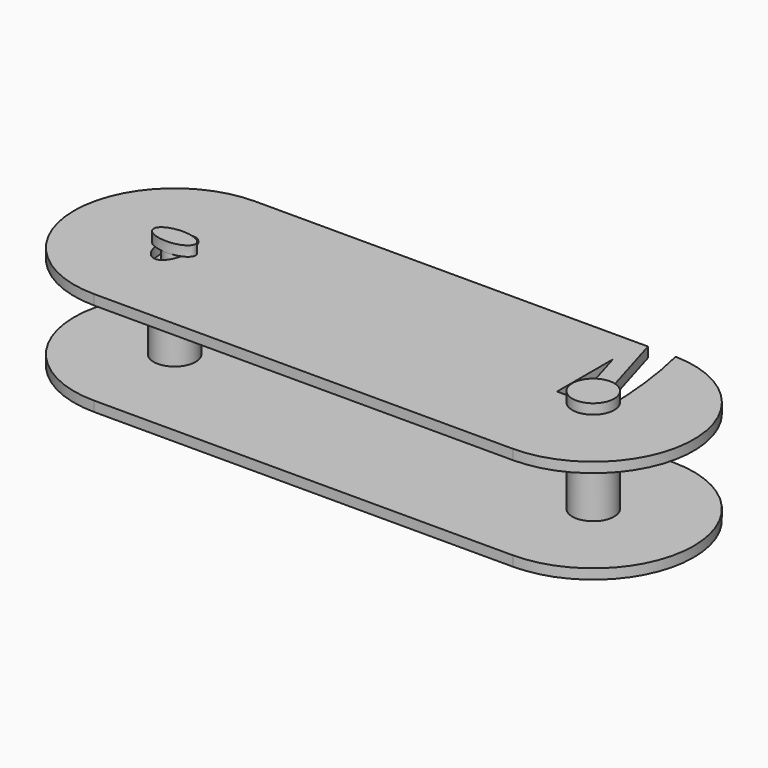
from build123d import *

# Parameters (mm, degrees)
F1_DEPTH  = 1.2
F2_R      = 2.5
F3_DEPTH  = 10
F4_R      = 1.25
F5_R      = 1.25
F6_DEPTH  = 1.2
F8_R      = 2.5
F8_R_2    = 1.25
F9_DEPTH  = 1.2
F11_DEPTH = 1.2


with BuildPart() as f1:
    # F0 (on Top) → F1 (new body)
    with BuildSketch(Plane.XY):
        with BuildLine():
            ThreePointArc((0, 12), (-12, 0), (0, -12))
            Line((0, -12), (50, -12))
            ThreePointArc((50, -12), (62, 0), (50, 12))
            Line((50, 12), (0, 12))
        make_face()
    extrude(amount=F1_DEPTH)

    # F2 (on face) → F3 (join)
    with BuildSketch(Plane.XY.offset(1.2)):
        Circle(F2_R)
        with Locations((50, 0)):
            Circle(F2_R)
    extrude(amount=F3_DEPTH)

    # F4 (on face) + F5 (on face) → F6 (join)
    with BuildSketch(Plane.XY.offset(11.2)):
        Circle(F4_R)
    with BuildSketch(Plane.XY.offset(11.2)):
        with Locations((50, 0)):
            Circle(F5_R)
    extrude(amount=F6_DEPTH)

    # F7 (on face) + F8 (on face) → F9 (join)
    with BuildSketch(Plane.XY.offset(12.4)):
        with BuildLine():
            add(Edge.make_bspline(
                [(4.2e-09, -1.25), (2.5000000021, -1.2499999979), (2.5, 1e-09), (2.4999999979, 1.25), (0, 1.25)],
                knots=[1.5707963285, 1.5707963285, 1.5707963285, 3.1415926544, 3.1415926544, 4.7123889804, 4.7123889804, 4.7123889804], degree=2, weights=[1, 0.7071067815, 1, 0.7071067815, 1]))
            ThreePointArc((0, 1.25), (0.8838834765, 0.8838834765), (1.25, 0))
            ThreePointArc((1.25, 0), (0.883883478, -0.883883475), (4.2e-09, -1.25))
        make_face()
        with BuildLine():
            ThreePointArc((1.25, 0), (0.8838834765, 0.8838834765), (0, 1.25))
            ThreePointArc((0, 1.25), (-1.25, -2.1e-09), (4.2e-09, -1.25))
            ThreePointArc((4.2e-09, -1.25), (0.883883478, -0.883883475), (1.25, 0))
        make_face()
        with BuildLine():
            ThreePointArc((4.2e-09, -1.25), (-1.25, -2.1e-09), (0, 1.25))
            add(Edge.make_bspline(
                [(0, 1.25), (-2.5000000021, 1.25), (-2.5, -1e-09), (-2.4999999979, -1.2500000021), (4.2e-09, -1.25)],
                knots=[4.7123889804, 4.7123889804, 4.7123889804, 6.283185308, 6.283185308, 7.8539816357, 7.8539816357, 7.8539816357], degree=2, weights=[1, 0.7071067809, 1, 0.7071067809, 1]))
        make_face()
    with BuildSketch(Plane.XY.offset(12.4)):
        with Locations((50, 0)):
            Circle(F8_R)
        with Locations((50, 0)):
            Circle(F8_R_2, mode=Mode.SUBTRACT)
        with Locations((50, 0)):
            Circle(F8_R_2)
    extrude(amount=F9_DEPTH)


with BuildPart() as f11:
    # F10 (on face) → F11 (new body)
    with BuildSketch(Plane.XY.offset(11.2)):
        with BuildLine():
            ThreePointArc((0, 12), (-12, 0), (0, -12))
            Line((0, -12), (50, -12))
            ThreePointArc((50, -12), (61.9994137232, -0.1186182953), (50.237225, 11.99765495))
            ThreePointArc((50.237225, 11.99765495), (51.2955903136, 6.0402743626), (51.65, 0))
            ThreePointArc((51.65, 0), (50.2015083771, -1.6376490387), (48.3992189406, -0.4))
            Line((48.3992189406, -0.4), (45.9992189406, -0.4))
            Line((45.9992189406, -0.4), (45.9992189406, 7.9439693035))
            Line((45.9992189406, 7.9439693035), (48.35, 0))
            ThreePointArc((48.35, 0), (48.833273811, 1.166726189), (50, 1.65))
            Line((50, 1.65), (46.9372258332, 12))
            Line((46.9372258332, 12), (0, 12))
        make_face()
        with BuildLine():
            add(Edge.make_bspline(
                [(1.0168341302, 2.2838669733), (0, 3.6823510732), (-1.0168341302, 2.2838669733)],
                knots=[5.6191964791, 5.6191964791, 5.6191964791, 6.9471741352, 6.9471741352, 6.9471741352], degree=2, weights=[1, 0.7875403356, 1]))
            ThreePointArc((1.0168341302, 2.2838669733), (2.0966741909, 1.3616010198), (2.5, 0))
            ThreePointArc((2.5, 0), (2.0966741909, -1.3616010198), (1.0168341302, -2.2838669733))
            add(Edge.make_bspline(
                [(-1.0168341302, -2.2838669733), (0, -3.6823510732), (1.0168341302, -2.2838669733)],
                knots=[2.4776038255, 2.4776038255, 2.4776038255, 3.8055814816, 3.8055814816, 3.8055814816], degree=2, weights=[1, 0.7875403356, 1]))
            ThreePointArc((-1.0168341302, -2.2838669733), (-2.5, 0), (-1.0168341302, 2.2838669733))
        make_face(mode=Mode.SUBTRACT)
        with BuildLine():
            add(Edge.make_bspline(
                [(1.65, 0), (1.65, 1.4130539516), (1.0168341302, 2.2838669733)],
                knots=[4.7123889804, 4.7123889804, 4.7123889804, 5.6191964791, 5.6191964791, 5.6191964791], degree=2, weights=[1, 0.8989613755, 1]))
            add(Edge.make_bspline(
                [(1.0168341302, -2.2838669733), (1.65, -1.4130539516), (1.65, 0)],
                knots=[3.8055814816, 3.8055814816, 3.8055814816, 4.7123889804, 4.7123889804, 4.7123889804], degree=2, weights=[1, 0.8989613755, 1]))
            ThreePointArc((1.0168341302, -2.2838669733), (2.0966741909, -1.3616010198), (2.5, 0))
            ThreePointArc((2.5, 0), (2.0966741909, 1.3616010198), (1.0168341302, 2.2838669733))
        make_face()
        with BuildLine():
            add(Edge.make_bspline(
                [(-1.0168341302, 2.2838669733), (-2.6774278313, 0), (-1.0168341302, -2.2838669733)],
                knots=[0.663988828, 0.663988828, 0.663988828, 2.4776038255, 2.4776038255, 2.4776038255], degree=2, weights=[1, 0.6162631092, 1]))
            ThreePointArc((-1.0168341302, 2.2838669733), (-2.5, 0), (-1.0168341302, -2.2838669733))
        make_face()
    extrude(amount=F11_DEPTH)


solid = Compound([f1.part, f11.part])
